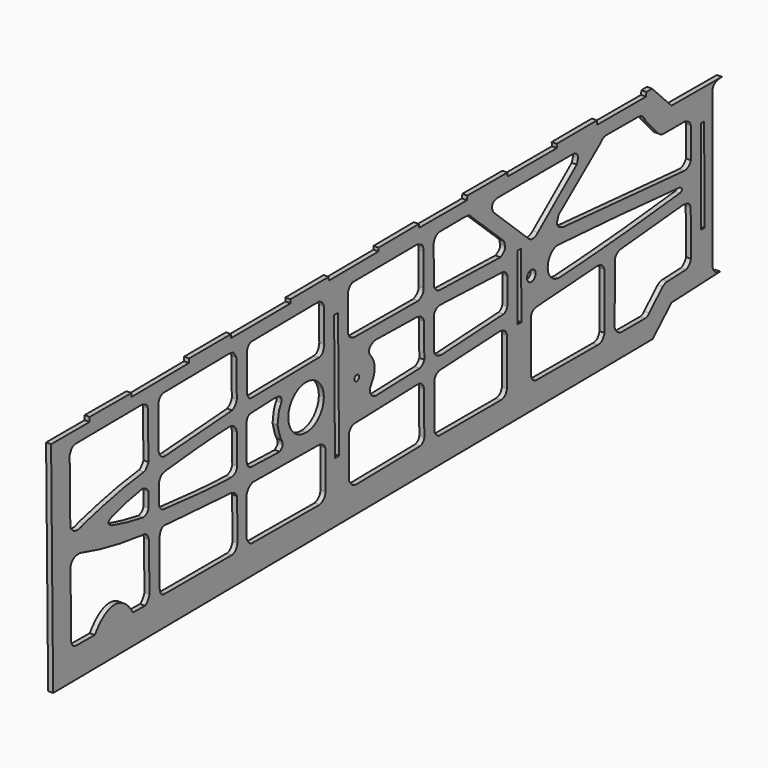
from build123d import *

# Parameters (mm, degrees)
F1_DEPTH = 3


# Not quite as in the source:
# - ends of sketch curves that miss each other by under 0.0002 mm in the source are joined


with BuildPart() as f1:
    # F0 (on Right) → F1 (new body)
    with BuildSketch(Plane.YZ):
        with BuildLine():
            Line((-223.454028, 63.686141), (-252.359227, 63.686134))
            Line((-252.359227, 63.686134), (-250.815738, -68.351794))
            Line((-250.815738, -68.351794), (198.741292, -64.166358))
            Line((198.741292, -64.166358), (212.947304, -50.654891))
            Line((212.947304, -50.654891), (249.3845559243, -49.0590650289))
            add(Edge.make_bspline(
                [(243.519284, -44.217356), (244.3534650538, -46.8721012451), (245.7624389816, -48.993112909), (249.3845559243, -49.0590650289)],
                knots=[0, 0, 0, 0, 0.8995873514, 0.8995873514, 0.8995873514, 0.8995873514], degree=3))
            Line((243.519284, -44.217356), (243.659587, 49.022967))
            add(Edge.make_bspline(
                [(250.7015376364, 53.2383428294), (246.4280040816, 53.1173614606), (243.8476255087, 51.8676123711), (243.659587, 49.022967)],
                knots=[0.1098221015, 0.1098221015, 0.1098221015, 0.1098221015, 1, 1, 1, 1], degree=3))
            Line((250.7015376364, 53.2383428294), (212.860117, 53.372772))
            Line((212.860117, 53.372772), (198.267202, 68.316484))
            Line((198.267202, 68.316484), (194.057707, 68.246359))
            Line((194.057707, 68.246359), (193.777087, 65.860969))
            Line((193.777087, 65.860969), (157.084319, 65.931169))
            Line((157.084319, 65.931169), (156.968077, 68.351794))
            Line((156.968077, 68.351794), (126.809999, 68.228509))
            Line((126.809999, 68.228509), (126.940349, 65.890062))
            Line((126.940349, 65.890062), (90.132194, 65.858937))
            Line((90.132194, 65.858937), (89.831609, 68.061207))
            Line((89.831609, 68.061207), (59.792714, 68.095257))
            Line((59.792714, 68.095257), (59.523254, 65.725692))
            Line((59.523254, 65.725692), (23.468969, 65.793792))
            Line((23.468969, 65.793792), (23.406719, 67.899747))
            Line((23.406719, 67.899747), (-6.771301, 67.670202))
            Line((-6.771301, 67.670202), (-6.808276, 65.663457))
            Line((-6.808276, 65.663457), (-44.109608, 65.433882))
            Line((-44.109608, 65.433882), (-44.211743, 67.471759))
            Line((-44.211743, 67.471759), (-72.867444, 67.273324))
            Line((-72.867444, 67.273324), (-72.768226, 65.068144))
            Line((-72.768226, 65.068144), (-117.241494, 64.866784))
            Line((-117.241494, 64.866784), (-117.471054, 67.006782))
            Line((-117.471054, 67.006782), (-148.805656, 66.913414))
            Line((-148.805656, 66.913414), (-149.016129, 64.528031))
            Line((-149.016129, 64.528031), (-192.093293, 64.107087))
            Line((-192.093293, 64.107087), (-192.093293, 66.211827))
            Line((-192.093293, 66.211827), (-223.45403, 66.352152))
            Line((-223.45403, 66.352152), (-223.454028, 63.686141))
        make_face()
        with BuildLine():
            add(Edge.make_bspline(
                [(-185.469361, -11.927434), (-183.188686, -12.714603), (-180.524828, -10.819504), (-178.966651, -16.664156)],
                knots=[0, 0, 0, 0, 1, 1, 1, 1], degree=3))
            Line((-178.966651, -16.664156), (-178.586798, -45.671486))
            add(Edge.make_bspline(
                [(-178.586798, -45.671486), (-179.367706, -47.536249), (-180.094936, -49.454689), (-181.903328, -50.291966)],
                knots=[0, 0, 0, 0, 1, 1, 1, 1], degree=3))
            Line((-181.903328, -50.291966), (-190.965773, -50.127559))
            add(Edge.make_bspline(
                [(-190.965773, -50.127559), (-197.718098, -38.522186), (-209.369941, -35.610289), (-219.624386, -50.391184)],
                knots=[0, 0, 0, 0, 1, 1, 1, 1], degree=3))
            Line((-219.624386, -50.391184), (-234.268371, -50.257916))
            add(Edge.make_bspline(
                [(-234.268371, -50.257916), (-236.57985, -49.769569), (-236.814172, -48.094279), (-237.352413, -46.592651)],
                knots=[0, 0, 0, 0, 1, 1, 1, 1], degree=3))
            Line((-237.352413, -46.592651), (-237.766312, -6.609506))
            add(Edge.make_bspline(
                [(-237.766312, -6.609506), (-236.873533, -4.170724), (-234.936552, -2.219291), (-230.370634, -2.666553)],
                knots=[0, 0, 0, 0, 1, 1, 1, 1], degree=3))
            add(Edge.make_bspline(
                [(-230.370634, -2.666553), (-215.684731, -7.300046), (-200.683981, -10.201894), (-185.469361, -11.927434)],
                knots=[0, 0, 0, 0, 1, 1, 1, 1], degree=3))
        make_face(mode=Mode.SUBTRACT)
        with BuildLine():
            add(Edge.make_bspline(
                [(-171.045819, -18.469173), (-170.595204, -15.154406), (-169.183906, -12.944419), (-165.012211, -13.908896)],
                knots=[0, 0, 0, 0, 1, 1, 1, 1], degree=3))
            Line((-165.012211, -13.908896), (-117.164289, -16.995858))
            add(Edge.make_bspline(
                [(-117.164289, -16.995858), (-115.697108, -17.654216), (-114.175929, -17.664588), (-112.884631, -20.433603)],
                knots=[0, 0, 0, 0, 1, 1, 1, 1], degree=3))
            Line((-112.884631, -20.433603), (-112.533834, -45.339799))
            add(Edge.make_bspline(
                [(-112.533834, -45.339799), (-113.115781, -47.830181), (-114.253869, -49.713858), (-116.883646, -49.970231)],
                knots=[0, 0, 0, 0, 1, 1, 1, 1], degree=3))
            Line((-116.883646, -49.970231), (-166.625843, -49.970231))
            add(Edge.make_bspline(
                [(-166.625843, -49.970231), (-170.627229, -50.111966), (-170.495881, -47.774058), (-170.905501, -45.760728)],
                knots=[0, 0, 0, 0, 1, 1, 1, 1], degree=3))
            Line((-170.905501, -45.760728), (-171.045819, -18.469173))
        make_face(mode=Mode.SUBTRACT)
        with BuildLine():
            add(Edge.make_bspline(
                [(-105.798646, -22.959304), (-105.402519, -20.674301), (-103.734421, -18.629246), (-101.098044, -17.837749)],
                knots=[0, 0, 0, 0, 1, 1, 1, 1], degree=3))
            Line((-101.098044, -17.837749), (-50.654259, -18.328856))
            add(Edge.make_bspline(
                [(-50.654259, -18.328856), (-48.908903, -19.015661), (-47.067421, -19.953596), (-46.708381, -22.026709)],
                knots=[0, 0, 0, 0, 1, 1, 1, 1], degree=3))
            Line((-46.708381, -22.026709), (-46.568063, -44.968459))
            add(Edge.make_bspline(
                [(-46.568063, -44.968459), (-46.795951, -46.929536), (-47.242666, -48.848539), (-50.847714, -50.160169)],
                knots=[0, 0, 0, 0, 1, 1, 1, 1], degree=3))
            Line((-50.847714, -50.160169), (-99.694876, -49.829906))
            add(Edge.make_bspline(
                [(-99.694876, -49.829906), (-102.242341, -50.413526), (-104.378469, -49.248956), (-105.868809, -45.339784)],
                knots=[0, 0, 0, 0, 1, 1, 1, 1], degree=3))
            Line((-105.868809, -45.339784), (-105.798646, -22.959304))
        make_face(mode=Mode.SUBTRACT)
        with BuildLine():
            add(Edge.make_bspline(
                [(-29.071021, -21.469594), (-28.403438, -20.100048), (-27.786834, -18.711394), (-25.663531, -17.887743)],
                knots=[0, 0, 0, 0, 1, 1, 1, 1], degree=3))
            Line((-25.663531, -17.887743), (22.464607, -16.416483))
            add(Edge.make_bspline(
                [(22.464607, -16.416483), (25.732439, -16.533971), (26.875619, -18.492821), (27.355394, -21.026628)],
                knots=[0, 0, 0, 0, 1, 1, 1, 1], degree=3))
            Line((27.355394, -21.026628), (27.507742, -46.520861))
            add(Edge.make_bspline(
                [(27.507742, -46.520861), (27.197144, -48.511601), (25.988241, -49.304599), (24.565222, -49.812101)],
                knots=[0, 0, 0, 0, 1, 1, 1, 1], degree=3))
            Line((24.565222, -49.812101), (-23.771326, -50.547731))
            add(Edge.make_bspline(
                [(-23.771326, -50.547731), (-26.975514, -50.091904), (-28.014856, -48.192844), (-29.024934, -46.274276)],
                knots=[0, 0, 0, 0, 1, 1, 1, 1], degree=3))
            Line((-29.024934, -46.274276), (-29.071021, -21.469594))
        make_face(mode=Mode.SUBTRACT)
        with BuildLine():
            add(Edge.make_bspline(
                [(34.990252, -19.272671), (35.928261, -16.636248), (37.734569, -15.881134), (39.786794, -15.658849)],
                knots=[0, 0, 0, 0, 1, 1, 1, 1], degree=3))
            Line((39.786794, -15.658849), (84.575549, -13.439921))
            add(Edge.make_bspline(
                [(84.575549, -13.439921), (86.447804, -14.186246), (88.551832, -13.773671), (89.722889, -18.025991)],
                knots=[0, 0, 0, 0, 1, 1, 1, 1], degree=3))
            Line((89.722889, -18.025991), (89.524447, -46.055899))
            add(Edge.make_bspline(
                [(89.524447, -46.055899), (88.801139, -47.715056), (88.813492, -49.646749), (84.972419, -50.150861)],
                knots=[0, 0, 0, 0, 1, 1, 1, 1], degree=3))
            Line((84.972419, -50.150861), (38.357489, -50.092736))
            add(Edge.make_bspline(
                [(38.357489, -50.092736), (37.293194, -49.510151), (36.228907, -48.673106), (35.164612, -46.975856)],
                knots=[0, 0, 0, 0, 1, 1, 1, 1], degree=3))
            Line((35.164612, -46.975856), (34.990252, -19.272671))
        make_face(mode=Mode.SUBTRACT)
        with BuildLine():
            add(Edge.make_bspline(
                [(107.395836, -16.614919), (107.336886, -13.966879), (108.337056, -11.933779), (112.356779, -11.653984)],
                knots=[0, 0, 0, 0, 1, 1, 1, 1], degree=3))
            Line((112.356779, -11.653984), (157.005216, -8.677421))
            add(Edge.make_bspline(
                [(157.005216, -8.677421), (161.068102, -8.682671), (161.816571, -10.713926), (162.595514, -12.726296)],
                knots=[0, 0, 0, 0, 1, 1, 1, 1], degree=3))
            Line((162.595514, -12.726296), (162.759899, -46.380544))
            add(Edge.make_bspline(
                [(162.759899, -46.380544), (161.656956, -48.155134), (161.504714, -50.523919), (157.600529, -50.547731)],
                knots=[0, 0, 0, 0, 1, 1, 1, 1], degree=3))
            Line((157.600529, -50.547731), (111.563024, -50.349296))
            add(Edge.make_bspline(
                [(111.563024, -50.349296), (109.135424, -50.263361), (108.270757, -48.614486), (107.594279, -46.777421)],
                knots=[0, 0, 0, 0, 1, 1, 1, 1], degree=3))
            Line((107.594279, -46.777421), (107.395836, -16.614919))
        make_face(mode=Mode.SUBTRACT)
        with BuildLine():
            add(Edge.make_bspline(
                [(170.569116, -10.880179), (170.618391, -8.514829), (172.438589, -7.920431), (173.906452, -6.973684)],
                knots=[0, 0, 0, 0, 1, 1, 1, 1], degree=3))
            Line((173.906452, -6.973684), (222.092714, -2.525861))
            add(Edge.make_bspline(
                [(222.092714, -2.525861), (224.573639, -2.888156), (227.001547, -3.316728), (227.286134, -6.424451)],
                knots=[0, 0, 0, 0, 1, 1, 1, 1], degree=3))
            Line((227.286134, -6.424451), (227.578806, -33.564304))
            add(Edge.make_bspline(
                [(227.578806, -33.564304), (226.806809, -35.571911), (225.586056, -36.951259), (223.878651, -37.649299)],
                knots=[0, 0, 0, 0, 1, 1, 1, 1], degree=3))
            Line((223.878651, -37.649299), (210.186464, -38.244611))
            add(Edge.make_bspline(
                [(210.186464, -38.244611), (208.760789, -37.950641), (207.521376, -38.774231), (206.277899, -39.573491)],
                knots=[0, 0, 0, 0, 1, 1, 1, 1], degree=3))
            Line((206.277899, -39.573491), (196.097399, -49.357106))
            add(Edge.make_bspline(
                [(196.097399, -49.357106), (195.487604, -50.554729), (194.205142, -50.631251), (193.064781, -50.944608)],
                knots=[0, 0, 0, 0, 1, 1, 1, 1], degree=3))
            Line((193.064781, -50.944608), (175.063026, -50.944608))
            add(Edge.make_bspline(
                [(175.063026, -50.944608), (172.519807, -50.312141), (170.878687, -48.777573), (170.206297, -46.274276)],
                knots=[0, 0, 0, 0, 1, 1, 1, 1], degree=3))
            Line((170.206297, -46.274276), (170.569116, -10.880179))
        make_face(mode=Mode.SUBTRACT)
        with BuildLine():
            add(Edge.make_bspline(
                [(-183.833708, 12.355819), (-181.731931, 11.665909), (-179.754391, 10.862119), (-179.213236, 8.741636)],
                knots=[0, 0, 0, 0, 1, 1, 1, 1], degree=3))
            Line((-179.213236, 8.741636), (-179.247286, 0.203494))
            add(Edge.make_bspline(
                [(-179.247286, 0.203494), (-179.772406, -1.527393), (-180.962356, -2.704263), (-183.074011, -3.113036)],
                knots=[0, 0, 0, 0, 1, 1, 1, 1], degree=3))
            add(Edge.make_bspline(
                [(-183.074011, -3.113036), (-190.995511, -1.719176), (-198.889996, -0.217271), (-206.550886, 2.218999)],
                knots=[0, 0, 0, 0, 1, 1, 1, 1], degree=3))
            add(Edge.make_bspline(
                [(-206.550886, 2.218999), (-211.698023, 4.504886), (-208.323691, 6.058902), (-206.601961, 6.972731)],
                knots=[0, 0, 0, 0, 1, 1, 1, 1], degree=3))
            add(Edge.make_bspline(
                [(-206.601961, 6.972731), (-198.882683, 9.416344), (-191.288401, 11.235034), (-183.833708, 12.355819)],
                knots=[0, 0, 0, 0, 1, 1, 1, 1], degree=3))
        make_face(mode=Mode.SUBTRACT)
        with BuildLine():
            add(Edge.make_bspline(
                [(-118.076341, 18.574392), (-115.710886, 18.018656), (-113.612281, 17.035961), (-113.095104, 13.522984)],
                knots=[0, 0, 0, 0, 1, 1, 1, 1], degree=3))
            Line((-113.095104, 13.522984), (-112.744314, -4.647994))
            add(Edge.make_bspline(
                [(-112.744314, -4.647994), (-113.135221, -6.587546), (-114.094824, -8.191879), (-117.023963, -8.787348)],
                knots=[0, 0, 0, 0, 1, 1, 1, 1], degree=3))
            add(Edge.make_bspline(
                [(-117.023963, -8.787348), (-133.428218, -8.425736), (-149.842133, -6.762558), (-166.255966, -5.110053)],
                knots=[0, 0, 0, 0, 1, 1, 1, 1], degree=3))
            add(Edge.make_bspline(
                [(-166.255966, -5.110053), (-169.180426, -5.151528), (-170.572659, -3.841008), (-171.255256, -1.904358)],
                knots=[0, 0, 0, 0, 1, 1, 1, 1], degree=3))
            Line((-171.255256, -1.904358), (-171.452236, 10.262081))
            add(Edge.make_bspline(
                [(-171.452236, 10.262081), (-170.768828, 13.413349), (-168.927143, 14.353347), (-166.801246, 14.750756)],
                knots=[0, 0, 0, 0, 1, 1, 1, 1], degree=3))
            add(Edge.make_bspline(
                [(-166.801246, 14.750756), (-150.402271, 16.392424), (-133.934971, 18.193526), (-118.076341, 18.574392)],
                knots=[0, 0, 0, 0, 1, 1, 1, 1], degree=3))
        make_face(mode=Mode.SUBTRACT)
        with BuildLine():
            add(Edge.make_bspline(
                [(-238.409774, 52.190149), (-237.500049, 54.070061), (-237.025687, 56.330929), (-234.101058, 56.447801)],
                knots=[0, 0, 0, 0, 1, 1, 1, 1], degree=3))
            Line((-234.101058, 56.447801), (-184.148393, 56.892821))
            add(Edge.make_bspline(
                [(-184.148393, 56.892821), (-182.244473, 56.194519), (-179.993078, 55.843692), (-179.856698, 53.377856)],
                knots=[0, 0, 0, 0, 1, 1, 1, 1], degree=3))
            Line((-179.856698, 53.377856), (-179.281328, 24.517879))
            add(Edge.make_bspline(
                [(-179.281328, 24.517879), (-180.728888, 22.004479), (-181.942906, 20.658784), (-182.861461, 20.790387)],
                knots=[0, 0, 0, 0, 1, 1, 1, 1], degree=3))
            add(Edge.make_bspline(
                [(-182.861461, 20.790387), (-197.639273, 19.169794), (-212.623171, 15.694362), (-227.663524, 11.710902)],
                knots=[0, 0, 0, 0, 1, 1, 1, 1], degree=3))
            add(Edge.make_bspline(
                [(-227.663524, 11.710902), (-231.857013, 9.781962), (-235.58942, 9.437554), (-237.930701, 13.873774)],
                knots=[0, 0, 0, 0, 1, 1, 1, 1], degree=3))
            Line((-237.930701, 13.873774), (-238.409774, 52.190149))
        make_face(mode=Mode.SUBTRACT)
        with BuildLine():
            add(Edge.make_bspline(
                [(-105.864181, 15.103309), (-105.561541, 16.600804), (-105.670156, 18.193212), (-103.040469, 19.153699)],
                knots=[0, 0, 0, 0, 1, 1, 1, 1], degree=3))
            Line((-103.040469, 19.153699), (-84.505629, 19.907382))
            add(Edge.make_bspline(
                [(-84.505629, 19.907382), (-81.843466, 19.715929), (-79.037169, 19.897256), (-79.734856, 15.347104)],
                knots=[0, 0, 0, 0, 1, 1, 1, 1], degree=3))
            add(Edge.make_bspline(
                [(-79.734856, 15.347104), (-81.852713, 12.369904), (-81.985329, 8.510374), (-82.506114, 4.823359)],
                knots=[0, 0, 0, 0, 1, 1, 1, 1], degree=3))
            add(Edge.make_bspline(
                [(-82.506114, 4.823359), (-81.551266, 1.417572), (-80.920584, -2.717599), (-79.278826, -4.577838)],
                knots=[0, 0, 0, 0, 1, 1, 1, 1], degree=3))
            add(Edge.make_bspline(
                [(-79.278826, -4.577838), (-79.135276, -6.197516), (-77.207634, -7.343171), (-80.892474, -9.980021)],
                knots=[0, 0, 0, 0, 1, 1, 1, 1], degree=3))
            Line((-80.892474, -9.980021), (-101.799624, -9.348611))
            add(Edge.make_bspline(
                [(-101.799624, -9.348611), (-105.385966, -8.766093), (-105.116416, -6.822678), (-105.703681, -5.181671)],
                knots=[0, 0, 0, 0, 1, 1, 1, 1], degree=3))
            Line((-105.703681, -5.181671), (-105.864181, 15.103309))
        make_face(mode=Mode.SUBTRACT)
        with BuildLine():
            add(Edge.make_bspline(
                [(-61.159628, 18.750199), (-53.802453, 18.750197), (-47.838285, 12.786026), (-47.838286, 5.428849)],
                knots=[0, 0, 0, 0, 1, 1, 1, 1], degree=3))
            add(Edge.make_bspline(
                [(-47.838286, 5.428849), (-47.838285, -1.928328), (-53.802453, -7.892499), (-61.159628, -7.892501)],
                knots=[0, 0, 0, 0, 1, 1, 1, 1], degree=3))
            add(Edge.make_bspline(
                [(-61.159628, -7.892501), (-64.69267, -7.892502), (-68.081008, -6.489007), (-70.579246, -3.990769)],
                knots=[0, 0, 0, 0, 1, 1, 1, 1], degree=3))
            add(Edge.make_bspline(
                [(-70.579246, -3.990769), (-73.077484, -1.492531), (-74.480979, 1.895807), (-74.480978, 5.428849)],
                knots=[0, 0, 0, 0, 1, 1, 1, 1], degree=3))
            add(Edge.make_bspline(
                [(-74.480978, 5.428849), (-74.480979, 8.961891), (-73.077484, 12.350229), (-70.579246, 14.848467)],
                knots=[0, 0, 0, 0, 1, 1, 1, 1], degree=3))
            add(Edge.make_bspline(
                [(-70.579246, 14.848467), (-68.081008, 17.346705), (-64.69267, 18.7502), (-61.159628, 18.750199)],
                knots=[0, 0, 0, 0, 1, 1, 1, 1], degree=3))
        make_face(mode=Mode.SUBTRACT)
        Polygon((-39.476949, -30.285199), (-40.121873, 45.641921), (-37.195644, 45.671097), (-36.372106, -30.251899), align=None, mode=Mode.SUBTRACT)
        with BuildLine():
            add(Edge.make_bspline(
                [(-21.900821, 6.686867), (-21.575981, 6.362028), (-21.393488, 5.921451), (-21.393488, 5.462059)],
                knots=[0, 0, 0, 0, 1, 1, 1, 1], degree=3))
            add(Edge.make_bspline(
                [(-21.393488, 5.462059), (-21.393488, 5.002667), (-21.575981, 4.56209), (-21.900821, 4.237251)],
                knots=[0, 0, 0, 0, 1, 1, 1, 1], degree=3))
            add(Edge.make_bspline(
                [(-21.900821, 4.237251), (-22.22566, 3.912412), (-22.666236, 3.729919), (-23.125628, 3.729919)],
                knots=[0, 0, 0, 0, 1, 1, 1, 1], degree=3))
            add(Edge.make_bspline(
                [(-23.125628, 3.729919), (-23.585021, 3.729919), (-24.025597, 3.912412), (-24.350436, 4.237251)],
                knots=[0, 0, 0, 0, 1, 1, 1, 1], degree=3))
            add(Edge.make_bspline(
                [(-24.350436, 4.237251), (-24.675276, 4.56209), (-24.857769, 5.002667), (-24.857769, 5.462059)],
                knots=[0, 0, 0, 0, 1, 1, 1, 1], degree=3))
            add(Edge.make_bspline(
                [(-24.857769, 5.462059), (-24.857769, 5.921451), (-24.675276, 6.362028), (-24.350436, 6.686867)],
                knots=[0, 0, 0, 0, 1, 1, 1, 1], degree=3))
            add(Edge.make_bspline(
                [(-24.350436, 6.686867), (-24.025597, 7.011706), (-23.585021, 7.194199), (-23.125628, 7.194199)],
                knots=[0, 0, 0, 0, 1, 1, 1, 1], degree=3))
            add(Edge.make_bspline(
                [(-23.125628, 7.194199), (-22.666236, 7.194199), (-22.22566, 7.011706), (-21.900821, 6.686867)],
                knots=[0, 0, 0, 0, 1, 1, 1, 1], degree=3))
        make_face(mode=Mode.SUBTRACT)
        with BuildLine():
            add(Edge.make_bspline(
                [(-171.817561, 52.951917), (-171.089573, 55.028696), (-169.970063, 56.744067), (-166.836324, 56.600149)],
                knots=[0, 0, 0, 0, 1, 1, 1, 1], degree=3))
            Line((-166.836324, 56.600149), (-118.567448, 57.231574))
            add(Edge.make_bspline(
                [(-118.567448, 57.231574), (-116.954214, 56.522877), (-115.773249, 58.234947), (-113.305584, 52.741444)],
                knots=[0, 0, 0, 0, 1, 1, 1, 1], degree=3))
            Line((-113.305584, 52.741444), (-113.095104, 30.641606))
            add(Edge.make_bspline(
                [(-113.095104, 30.641606), (-113.535286, 29.269339), (-113.743569, 27.914907), (-116.532856, 26.361942)],
                knots=[0, 0, 0, 0, 1, 1, 1, 1], degree=3))
            Line((-116.532856, 26.361942), (-165.854109, 22.783879))
            add(Edge.make_bspline(
                [(-165.854109, 22.783879), (-169.567996, 22.390804), (-170.932643, 24.346984), (-171.677244, 26.923204)],
                knots=[0, 0, 0, 0, 1, 1, 1, 1], degree=3))
            Line((-171.677244, 26.923204), (-171.817561, 52.951917))
        make_face(mode=Mode.SUBTRACT)
        with BuildLine():
            add(Edge.make_bspline(
                [(-105.488956, 53.346739), (-104.721406, 55.440896), (-103.615276, 56.857879), (-101.792574, 56.841739)],
                knots=[0, 0, 0, 0, 1, 1, 1, 1], degree=3))
            Line((-101.792574, 56.841739), (-51.426016, 57.371884))
            add(Edge.make_bspline(
                [(-51.426016, 57.371884), (-49.652019, 56.577754), (-48.227049, 55.481134), (-47.847931, 53.478102)],
                knots=[0, 0, 0, 0, 1, 1, 1, 1], degree=3))
            Line((-47.847931, 53.478102), (-47.497149, 32.956812))
            add(Edge.make_bspline(
                [(-47.497149, 32.956812), (-47.938929, 30.634249), (-48.416206, 28.099399), (-51.443019, 27.823227)],
                knots=[0, 0, 0, 0, 1, 1, 1, 1], degree=3))
            Line((-51.443019, 27.823227), (-100.817409, 27.063537))
            add(Edge.make_bspline(
                [(-100.817409, 27.063537), (-104.610886, 26.583717), (-104.464771, 28.969062), (-105.588174, 30.431119)],
                knots=[0, 0, 0, 0, 1, 1, 1, 1], degree=3))
            Line((-105.588174, 30.431119), (-105.488956, 53.346739))
        make_face(mode=Mode.SUBTRACT)
        with BuildLine():
            add(Edge.make_bspline(
                [(-29.774063, 53.532732), (-29.035883, 54.940324), (-28.471073, 56.405697), (-26.202189, 57.303049)],
                knots=[0, 0, 0, 0, 1, 1, 1, 1], degree=3))
            Line((-26.202189, 57.303049), (22.514219, 57.600701))
            add(Edge.make_bspline(
                [(22.514219, 57.600701), (24.302279, 56.412409), (26.891234, 56.997544), (26.979067, 52.044454)],
                knots=[0, 0, 0, 0, 1, 1, 1, 1], degree=3))
            Line((26.979067, 52.044454), (27.028642, 32.597577))
            add(Edge.make_bspline(
                [(27.028642, 32.597577), (27.078667, 29.990074), (25.430242, 28.514824), (23.109501, 27.487811)],
                knots=[0, 0, 0, 0, 1, 1, 1, 1], degree=3))
            Line((23.109501, 27.487811), (-25.061199, 27.785464))
            add(Edge.make_bspline(
                [(-25.061199, 27.785464), (-29.408139, 28.825721), (-28.783726, 30.398622), (-29.724481, 31.803829)],
                knots=[0, 0, 0, 0, 1, 1, 1, 1], degree=3))
            Line((-29.724481, 31.803829), (-29.774063, 53.532732))
        make_face(mode=Mode.SUBTRACT)
        with BuildLine():
            add(Edge.make_bspline(
                [(-13.452578, 13.944454), (-14.252011, 16.065911), (-14.415826, 18.144986), (-9.682261, 19.897579)],
                knots=[0, 0, 0, 0, 1, 1, 1, 1], degree=3))
            Line((-9.682261, 19.897579), (22.067736, 19.302267))
            add(Edge.make_bspline(
                [(22.067736, 19.302267), (24.587421, 18.748256), (26.777024, 17.804141), (27.261156, 14.844469)],
                knots=[0, 0, 0, 0, 1, 1, 1, 1], degree=3))
            Line((27.261156, 14.844469), (27.524766, -5.452811))
            add(Edge.make_bspline(
                [(27.524766, -5.452811), (26.843436, -7.085636), (25.709076, -8.135988), (24.101721, -8.578204)],
                knots=[0, 0, 0, 0, 1, 1, 1, 1], degree=3))
            Line((24.101721, -8.578204), (-8.690071, -9.669611))
            add(Edge.make_bspline(
                [(-8.690071, -9.669611), (-11.914981, -9.472414), (-13.932293, -6.572231), (-13.105314, -3.716486)],
                knots=[0, 0, 0, 0, 1, 1, 1, 1], degree=3))
            add(Edge.make_bspline(
                [(-13.105314, -3.716486), (-11.293246, -0.554546), (-10.178266, 0.797921), (-9.682261, 4.617889)],
                knots=[0, 0, 0, 0, 1, 1, 1, 1], degree=3))
            add(Edge.make_bspline(
                [(-9.682261, 4.617889), (-9.536611, 8.895432), (-11.388211, 11.508596), (-13.452578, 13.944454)],
                knots=[0, 0, 0, 0, 1, 1, 1, 1], degree=3))
        make_face(mode=Mode.SUBTRACT)
        with BuildLine():
            add(Edge.make_bspline(
                [(34.779771, 15.509944), (35.615227, 17.153539), (36.827384, 18.357656), (38.782566, 18.694917)],
                knots=[0, 0, 0, 0, 1, 1, 1, 1], degree=3))
            Line((38.782566, 18.694917), (86.700239, 16.908979))
            add(Edge.make_bspline(
                [(86.700239, 16.908979), (88.460699, 16.129654), (89.598487, 14.961161), (89.863207, 13.246999)],
                knots=[0, 0, 0, 0, 1, 1, 1, 1], degree=3))
            Line((89.863207, 13.246999), (89.781007, -2.610116))
            add(Edge.make_bspline(
                [(89.781007, -2.610116), (89.221551, -4.311101), (88.273964, -5.106431), (87.155234, -5.502423)],
                knots=[0, 0, 0, 0, 1, 1, 1, 1], degree=3))
            Line((87.155234, -5.502423), (40.522424, -8.082108))
            add(Edge.make_bspline(
                [(40.522424, -8.082108), (37.296959, -7.879676), (35.373959, -6.560853), (34.767734, -4.113356)],
                knots=[0, 0, 0, 0, 1, 1, 1, 1], degree=3))
            Line((34.767734, -4.113356), (34.779771, 15.509944))
        make_face(mode=Mode.SUBTRACT)
        Polygon((97.275516, -15.225858), (97.415864, 23.689901), (100.181931, 23.830219), (100.252056, -15.225858), align=None, mode=Mode.SUBTRACT)
        with BuildLine():
            add(Edge.make_bspline(
                [(110.077251, 8.489898), (110.679818, 7.887331), (111.018337, 7.070075), (111.018337, 6.217917)],
                knots=[0, 0, 0, 0, 1, 1, 1, 1], degree=3))
            add(Edge.make_bspline(
                [(111.018337, 6.217917), (111.018337, 5.365758), (110.679818, 4.548502), (110.077251, 3.945935)],
                knots=[0, 0, 0, 0, 1, 1, 1, 1], degree=3))
            add(Edge.make_bspline(
                [(110.077251, 3.945935), (109.474684, 3.343368), (108.657428, 3.004849), (107.805269, 3.004849)],
                knots=[0, 0, 0, 0, 1, 1, 1, 1], degree=3))
            add(Edge.make_bspline(
                [(107.805269, 3.004849), (106.95311, 3.004849), (106.135854, 3.343368), (105.533287, 3.945935)],
                knots=[0, 0, 0, 0, 1, 1, 1, 1], degree=3))
            add(Edge.make_bspline(
                [(105.533287, 3.945935), (104.93072, 4.548502), (104.592201, 5.365758), (104.592202, 6.217916)],
                knots=[0, 0, 0, 0, 1, 1, 1, 1], degree=3))
            add(Edge.make_bspline(
                [(104.592202, 6.217916), (104.592201, 7.070075), (104.93072, 7.887331), (105.533287, 8.489898)],
                knots=[0, 0, 0, 0, 1, 1, 1, 1], degree=3))
            add(Edge.make_bspline(
                [(105.533287, 8.489898), (106.135854, 9.092465), (106.95311, 9.430984), (107.805269, 9.430984)],
                knots=[0, 0, 0, 0, 1, 1, 1, 1], degree=3))
            add(Edge.make_bspline(
                [(107.805269, 9.430984), (108.657428, 9.430984), (109.474684, 9.092465), (110.077251, 8.489898)],
                knots=[0, 0, 0, 0, 1, 1, 1, 1], degree=3))
        make_face(mode=Mode.SUBTRACT)
        with BuildLine():
            add(Edge.make_bspline(
                [(128.350087, -3.319608), (116.623139, -1.680648), (118.358257, 13.343202), (127.355827, 14.445537)],
                knots=[0, 0, 0, 0, 1, 1, 1, 1], degree=3))
            add(Edge.make_bspline(
                [(127.355827, 14.445537), (158.188192, 12.805114), (188.814217, 10.133029), (219.466941, 7.594452)],
                knots=[0, 0, 0, 0, 1, 1, 1, 1], degree=3))
            add(Edge.make_bspline(
                [(219.466941, 7.594452), (220.604399, 6.664804), (221.654946, 5.730581), (219.314587, 4.617889)],
                knots=[0, 0, 0, 0, 1, 1, 1, 1], degree=3))
            add(Edge.make_bspline(
                [(219.314587, 4.617889), (188.993084, 1.165054), (158.671582, -1.549983), (128.350087, -3.319608)],
                knots=[0, 0, 0, 0, 1, 1, 1, 1], degree=3))
        make_face(mode=Mode.SUBTRACT)
        Polygon((235.189589, -21.209643), (235.090364, 35.078044), (237.372397, 35.078044), (237.628956, -21.279768), align=None, mode=Mode.SUBTRACT)
        with BuildLine():
            add(Edge.make_bspline(
                [(34.569299, 53.036644), (34.976616, 55.562802), (36.554549, 56.764587), (38.538044, 57.451879)],
                knots=[0, 0, 0, 0, 1, 1, 1, 1], degree=3))
            Line((38.538044, 57.451879), (57.786486, 57.600701))
            add(Edge.make_bspline(
                [(57.786486, 57.600701), (59.853404, 57.406684), (62.020071, 57.426424), (63.193904, 55.318676)],
                knots=[0, 0, 0, 0, 1, 1, 1, 1], degree=3))
            Line((63.193904, 55.318676), (87.304056, 32.944841))
            add(Edge.make_bspline(
                [(87.304056, 32.944841), (87.731646, 30.476284), (89.988321, 28.046644), (84.575549, 25.453826)],
                knots=[0, 0, 0, 0, 1, 1, 1, 1], degree=3))
            Line((84.575549, 25.453826), (38.835704, 26.644459))
            add(Edge.make_bspline(
                [(38.835704, 26.644459), (35.136914, 27.712571), (35.834241, 28.989731), (34.668516, 30.117109)],
                knots=[0, 0, 0, 0, 1, 1, 1, 1], degree=3))
            Line((34.668516, 30.117109), (34.569299, 53.036644))
        make_face(mode=Mode.SUBTRACT)
        with BuildLine():
            add(Edge.make_bspline(
                [(79.217737, 51.449142), (77.700359, 54.622834), (77.883262, 57.078627), (82.293517, 57.749531)],
                knots=[0, 0, 0, 0, 1, 1, 1, 1], degree=3))
            Line((82.293517, 57.749531), (138.748964, 57.848749))
            add(Edge.make_bspline(
                [(138.748964, 57.848749), (142.108694, 57.552222), (143.867796, 55.928359), (141.824751, 51.151489)],
                knots=[0, 0, 0, 0, 1, 1, 1, 1], degree=3))
            Line((141.824751, 51.151489), (112.654431, 27.090941))
            add(Edge.make_bspline(
                [(112.654431, 27.090941), (109.409204, 24.434546), (107.195196, 25.284266), (105.262634, 27.090934)],
                knots=[0, 0, 0, 0, 1, 1, 1, 1], degree=3))
            Line((105.262634, 27.090934), (79.217737, 51.449142))
        make_face(mode=Mode.SUBTRACT)
        with BuildLine():
            add(Edge.make_bspline(
                [(131.803656, 22.278806), (124.739054, 24.133639), (127.550781, 27.262826), (128.231781, 30.117086)],
                knots=[0, 0, 0, 0, 1, 1, 1, 1], degree=3))
            Line((128.231781, 30.117086), (159.783337, 55.318676))
            add(Edge.make_bspline(
                [(159.783337, 55.318676), (160.756289, 56.462389), (161.744669, 57.590674), (163.752089, 57.699926)],
                knots=[0, 0, 0, 0, 1, 1, 1, 1], degree=3))
            Line((163.752089, 57.699926), (186.770841, 57.600701))
            add(Edge.make_bspline(
                [(186.770841, 57.600701), (190.117394, 57.838316), (192.137609, 56.292019), (193.120837, 53.731174)],
                knots=[0, 0, 0, 0, 1, 1, 1, 1], degree=3))
            Line((193.120837, 53.731174), (203.042714, 42.618679))
            add(Edge.make_bspline(
                [(203.042714, 42.618679), (204.262349, 41.899361), (205.056666, 40.885601), (207.408337, 40.950004)],
                knots=[0, 0, 0, 0, 1, 1, 1, 1], degree=3))
            Line((207.408337, 40.950004), (223.283339, 40.931929))
            add(Edge.make_bspline(
                [(223.283339, 40.931929), (225.152421, 40.177496), (226.935606, 39.300364), (227.518619, 36.708686)],
                knots=[0, 0, 0, 0, 1, 1, 1, 1], degree=3))
            Line((227.518619, 36.708686), (227.566769, 18.528439))
            add(Edge.make_bspline(
                [(227.566769, 18.528439), (226.485411, 16.786279), (225.305646, 15.142527), (222.571791, 15.052856)],
                knots=[0, 0, 0, 0, 1, 1, 1, 1], degree=3))
            Line((222.571791, 15.052856), (131.803656, 22.278806))
        make_face(mode=Mode.SUBTRACT)
    extrude(amount=F1_DEPTH)


solid = f1.part
